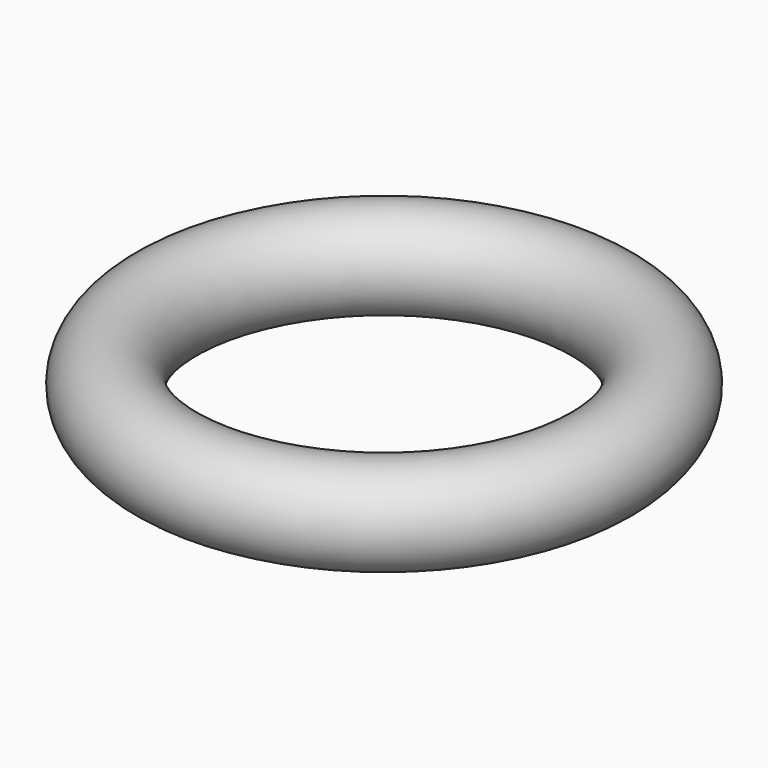
from build123d import *

# Parameters (mm, degrees)
F1_R = 4.3560693356


# Not quite as in the source:
# - the program builds the solid bodies; features that only make, move or delete a surface that nothing else refers to are left out


with BuildPart() as f3:
    # F1 (on Front) → F3 (revolve)
    with BuildSketch(Plane.XZ):
        with Locations((20.2592387795, 4.6241418459)):
            Circle(F1_R)
    revolve(axis=Axis((0, 0, 0.2561435103), (0, 0, -1)))


solid = f3.part
